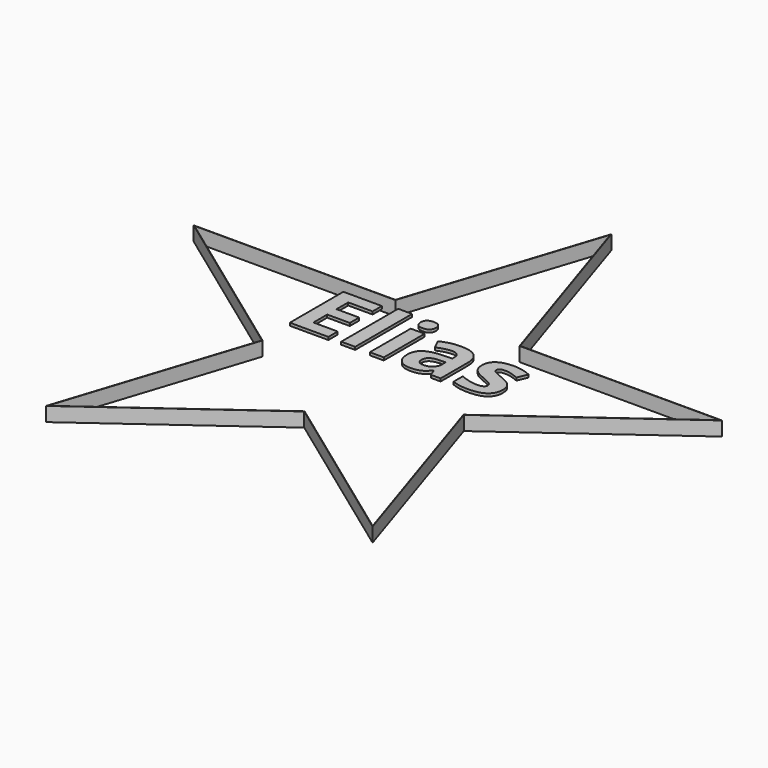
from build123d import *

# Parameters (mm, degrees)
F2_DEPTH     = 2.05
F3_TEXT_SIZE = 13.4940407853
F4_DEPTH     = 0.4


# Not quite as in the source:
# - Text() gives the source's letters only with a copy of the font that has no kerning and outlines rounded to 1/6400 em; it was checked with that copy


with BuildPart() as f2:
    # F1 (on Top) → F2 (new body)
    with BuildSketch(Plane.XY):
        Polygon((8.9805595316, 12.360679775), (0, 40), (-8.9805595316, 12.360679775), (-38.0422606518, 12.360679775), (-14.5308505601, -4.72135955), (-23.5114100917, -32.360679775), (0, -15.27864045), (23.5114100917, -32.360679775), (14.5308505601, -4.72135955), (38.0422606518, 12.360679775), align=None)
        Polygon((-14.4720720349, -4.7022612494), (-37.8883764749, 12.310679775), (-8.9442324052, 12.310679775), (0, 39.8381966011), (8.9442324052, 12.310679775), (37.8883764749, 12.310679775), (14.4720720349, -4.7022612494), (23.4163044401, -32.2297780756), (0, -15.2168370511), (-23.4163044401, -32.2297780756), align=None, mode=Mode.SUBTRACT)
    extrude(amount=F2_DEPTH)


with BuildPart() as f4:
    # F3 (on face) → F4 (new body)
    with BuildSketch(Plane.XY.offset(2.05)):
        with Locations((-15.5065504618, 0)):
            Text('Elias', F3_TEXT_SIZE, font='Open Sans', font_style=FontStyle.BOLD, text_align=(TextAlign.LEFT, TextAlign.BOTTOM))
    extrude(amount=F4_DEPTH)


solid = Compound([f2.part, f4.part])
